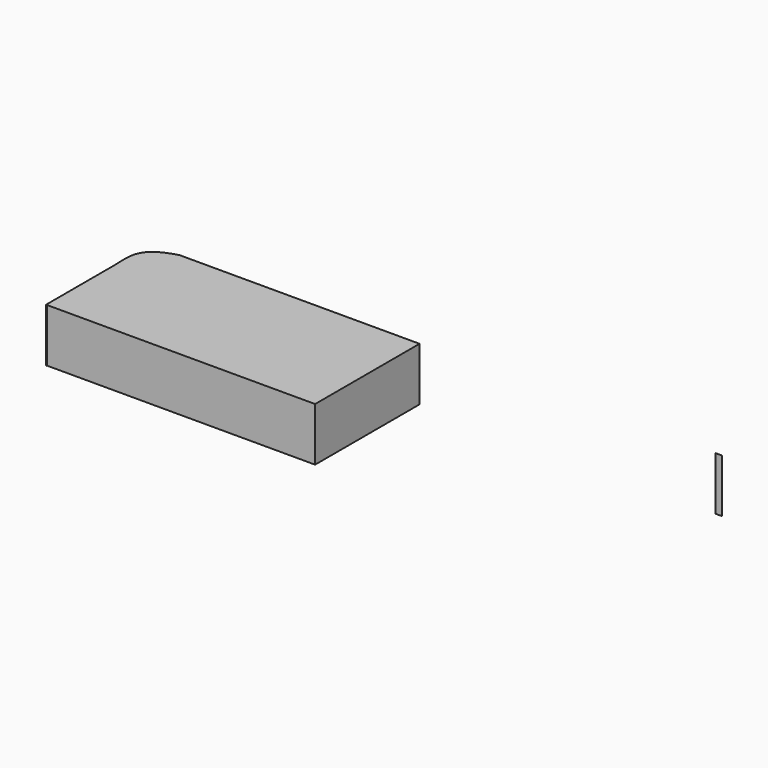
from build123d import *

# Parameters (mm, degrees)
F1_DEPTH = 9.906


with BuildPart() as f1:
    # F0 (on Top) → F1 (new body)
    with BuildSketch(Plane.XY):
        with BuildLine():
            Line((-10.4312598705, 35.8004160225), (-54.9399480224, 35.8004160225))
            add(Edge.make_bspline(
                [(-60.3583976626, 31.0863752262), (-60.0809005567, 33.179664896), (-58.9169910224, 34.7130967666), (-54.9399480224, 35.8004160225)],
                knots=[0.0210718605, 0.0210718605, 0.0210718605, 0.0210718605, 0.064974513, 0.064974513, 0.064974513, 0.064974513], degree=3))
            Line((-60.3583976626, 31.0863752262), (-60.3583976626, 27.6727415621))
            add(Edge.make_bspline(
                [(-60.1485681557, 11.5760835991), (-60.0368279013, 17.3156575533), (-60.1461253425, 23.3191062374), (-60.3583976626, 27.6727415621)],
                knots=[0.9280610246, 0.9280610246, 0.9280610246, 0.9280610246, 1, 1, 1, 1], degree=3))
            Line((-60.1485681557, 11.5760835991), (-10.4312598705, 11.5760835991))
            Line((-10.4312598705, 11.5760835991), (-10.4312598705, 35.8004160225))
        make_face()
        with BuildLine():
            Line((-60.3583976626, 27.6727415621), (-60.3583976626, 31.0863752262))
            add(Edge.make_bspline(
                [(-60.3583976626, 27.6727415621), (-60.4205749831, 28.9479779122), (-60.4915873444, 30.0816635409), (-60.3583976626, 31.0863752262)],
                knots=[0, 0, 0, 0, 0.0210718605, 0.0210718605, 0.0210718605, 0.0210718605], degree=3))
        make_face()
        with BuildLine():
            add(Edge.make_bspline(
                [(-60.1485681557, 11.5760835991), (-60.0368279013, 17.3156575533), (-60.1461253425, 23.3191062374), (-60.3583976626, 27.6727415621)],
                knots=[0.9280610246, 0.9280610246, 0.9280610246, 0.9280610246, 1, 1, 1, 1], degree=3))
            Line((-60.3583976626, 27.6727415621), (-60.3583976626, 11.5760835991))
            Line((-60.3583976626, 11.5760835991), (-60.1485681557, 11.5760835991))
        make_face()
        with BuildLine():
            add(Edge.make_bspline(
                [(-60.1508035203, 11.4627758061), (-60.1500487989, 11.500533273), (-60.1493036885, 11.5383027192), (-60.1485681557, 11.5760835991)],
                knots=[0.9275874847, 0.9275874847, 0.9275874847, 0.9275874847, 0.9280610246, 0.9280610246, 0.9280610246, 0.9280610246], degree=3))
            Line((-60.1485681557, 11.5760835991), (-60.3583976626, 11.5760835991))
            Line((-60.3583976626, 11.5760835991), (-60.1508035203, 11.4627758061))
        make_face()
    extrude(amount=F1_DEPTH)


with BuildPart() as f1b:
    # F0 (on Top) → F1, piece 2 (new body)
    with BuildSketch(Plane.XY):
        with BuildLine():
            add(Edge.make_bspline(
                [(45.6883870065, 35.8004160225), (45.6449263149, 35.7821790971), (45.2050634069, 35.7860902012), (44.5267579401, 35.8004160225)],
                knots=[0.2735171284, 0.2735171284, 0.2735171284, 0.2735171284, 0.2879295785, 0.2879295785, 0.2879295785, 0.2879295785], degree=3))
            Line((45.6883870065, 35.8004160225), (44.5267579401, 35.8004160225))
        make_face()
    extrude(amount=F1_DEPTH)


solid = Compound([f1.part, f1b.part])
